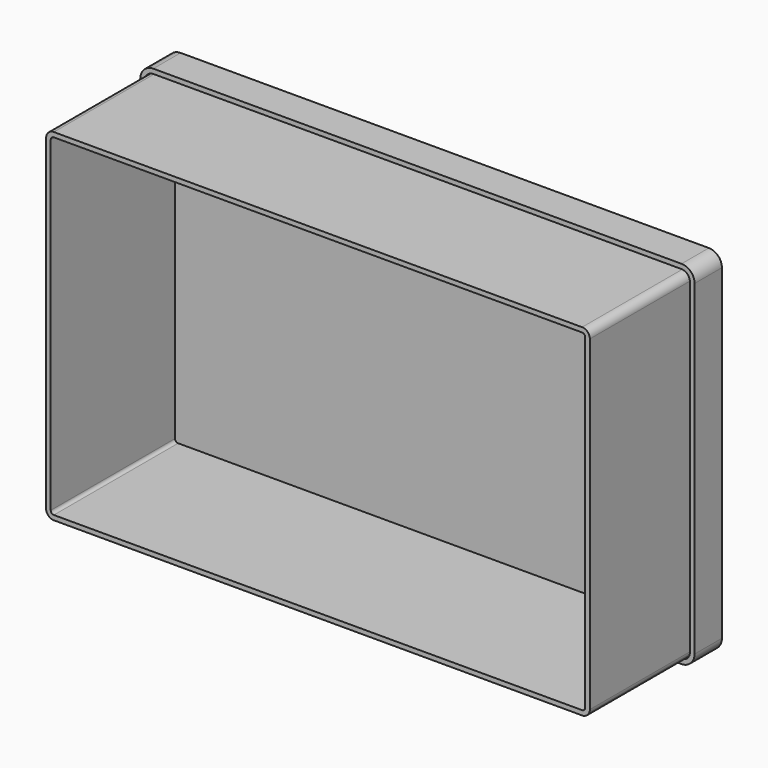
from build123d import *

# Parameters (mm, degrees)
F3_DEPTH = 50
F5_DEPTH = 10
F7_DEPTH = 1


with BuildPart() as f3:
    # F2 (on Front) → F3 (new body)
    with BuildSketch(Plane.XZ):
        with BuildLine():
            Line((87.5, -52.5), (87.5, 52.5))
            ThreePointArc((87.5, 52.5), (86.767766953, 54.267766953), (85, 55))
            Line((85, 55), (-85, 55))
            ThreePointArc((-85, 55), (-86.767766953, 54.267766953), (-87.5, 52.5))
            Line((-87.5, 52.5), (-87.5, -52.5))
            ThreePointArc((-87.5, -52.5), (-86.767766953, -54.267766953), (-85, -55))
            Line((-85, -55), (85, -55))
            ThreePointArc((85, -55), (86.767766953, -54.267766953), (87.5, -52.5))
        make_face()
        with BuildLine():
            ThreePointArc((-86, 52.5), (-85.7071067812, 53.2071067812), (-85, 53.5))
            Line((-85, 53.5), (85, 53.5))
            ThreePointArc((85, 53.5), (85.7071067812, 53.2071067812), (86, 52.5))
            Line((86, 52.5), (86, -52.5))
            ThreePointArc((86, -52.5), (85.7071067812, -53.2071067812), (85, -53.5))
            Line((85, -53.5), (-85, -53.5))
            ThreePointArc((-85, -53.5), (-85.7071067812, -53.2071067812), (-86, -52.5))
            Line((-86, -52.5), (-86, 52.5))
        make_face(mode=Mode.SUBTRACT)
    extrude(amount=F3_DEPTH)


with BuildPart() as f5:
    # F4 (on Front) → F5 (new body)
    with BuildSketch(Plane.XZ):
        with BuildLine():
            ThreePointArc((-89.2, -52.5), (-87.969848481, -55.469848481), (-85, -56.7))
            Line((-85, -56.7), (85, -56.7))
            ThreePointArc((85, -56.7), (87.969848481, -55.469848481), (89.2, -52.5))
            Line((89.2, -52.5), (89.2, 52.5))
            ThreePointArc((89.2, 52.5), (87.969848481, 55.469848481), (85, 56.7))
            Line((85, 56.7), (-85, 56.7))
            ThreePointArc((-85, 56.7), (-87.969848481, 55.469848481), (-89.2, 52.5))
            Line((-89.2, 52.5), (-89.2, -52.5))
        make_face()
        with BuildLine():
            Line((85, -55.2), (-85, -55.2))
            ThreePointArc((-85, -55.2), (-86.9091883092, -54.4091883092), (-87.7, -52.5))
            Line((-87.7, -52.5), (-87.7, 52.5))
            ThreePointArc((-87.7, 52.5), (-86.9091883092, 54.4091883092), (-85, 55.2))
            Line((-85, 55.2), (85, 55.2))
            ThreePointArc((85, 55.2), (86.9091883092, 54.4091883092), (87.7, 52.5))
            Line((87.7, 52.5), (87.7, -52.5))
            ThreePointArc((87.7, -52.5), (86.9091883092, -54.4091883092), (85, -55.2))
        make_face(mode=Mode.SUBTRACT)
    extrude(amount=F5_DEPTH)

    # F6 (on face) → F7 (join)
    with BuildSketch(Plane(origin=(0, 0, 0), x_dir=(-1, 0, 0), z_dir=(0, 1, 0))):
        with BuildLine():
            ThreePointArc((-85, 56.7), (-87.969848481, 55.469848481), (-89.2, 52.5))
            Line((-89.2, 52.5), (-89.2, -52.5))
            ThreePointArc((-89.2, -52.5), (-87.969848481, -55.469848481), (-85, -56.7))
            Line((-85, -56.7), (85, -56.7))
            ThreePointArc((85, -56.7), (87.969848481, -55.469848481), (89.2, -52.5))
            Line((89.2, -52.5), (89.2, 52.5))
            ThreePointArc((89.2, 52.5), (87.969848481, 55.469848481), (85, 56.7))
            Line((85, 56.7), (-85, 56.7))
        make_face()
    extrude(amount=F7_DEPTH)


solid = Compound([f3.part, f5.part])
